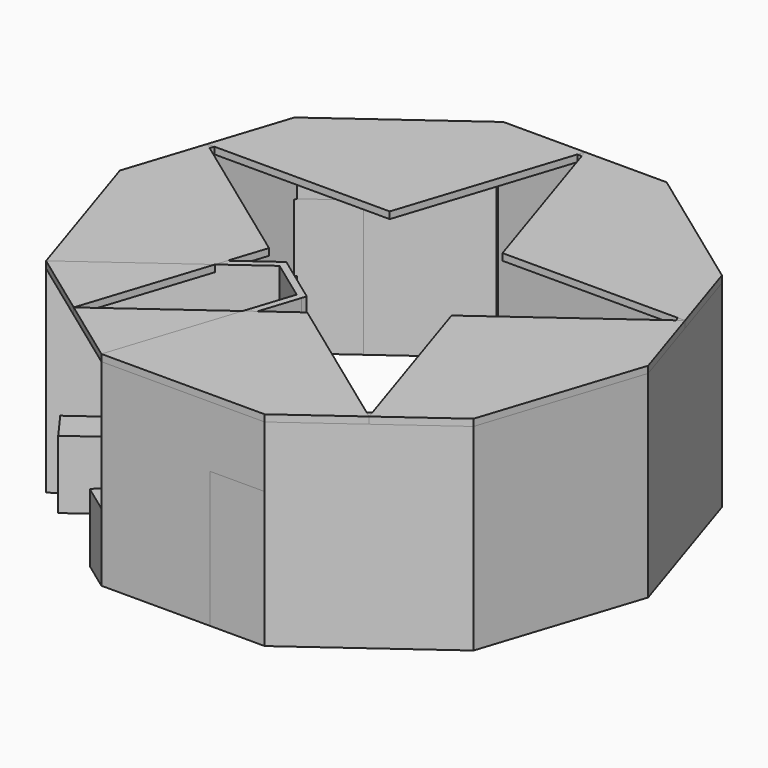
from build123d import *

# Parameters (mm, degrees)
F1_DEPTH     = 29.9999993294
F4_DEPTH     = 30
F6_DEPTH     = 10
F7_DEPTH     = 5
F9_DEPTH     = 30
F10_T        = 1
F10_T3_DEPTH = 32
F11_W        = 8
F11_H        = 20
F12_DEPTH    = 1.2370679775
F13_W        = 24
F13_H        = 10
F14_DEPTH    = 1.2370679775
F15_DEPTH    = 1
F17_DEPTH    = 1.2370679775
F18_DEPTH    = 1
F19_W        = 24
F19_H        = 29.9999993294
F20_DEPTH    = 1.2370679775
F21_DEPTH    = 1
F22_W        = 24
F22_H        = 10
F23_DEPTH    = 1.2370679775
F24_DEPTH    = 1
F25_DEPTH    = 1
F26_DEPTH    = 1
F28_DEPTH    = 1
F30_DEPTH    = 1
F31_DEPTH    = 1
F33_DEPTH    = 1
F34_DEPTH    = 10


# Not quite as in the source:
# - a shell that OpenCascade refuses in one call is made with other operations: the cavity is built on its own and cut out


with BuildPart() as f1:
    # F0 (on Top) → F1 (new body)
    with BuildSketch(Plane.XY):
        Polygon((31.416407865, 22.8253563911), (12, 36.9322024461), (-12, 36.9322024461), (-31.416407865, 22.8253563911), (-38.83281573, 0), (-31.416407865, -22.8253563911), (-12, -36.9322024461), (12, -36.9322024461), (31.416407865, -22.8253563911), (38.83281573, 0), align=None)
    extrude(amount=-F1_DEPTH)

    # F3 (on face) → F4 (cut)
    with BuildSketch(Plane.XY):
        Polygon((0, 0), (-31.416407865, -22.8253563911), (-12, -36.9322024461), align=None)
    extrude(amount=-F4_DEPTH, mode=Mode.SUBTRACT)

    # F8 (on face) → F9 (join)
    with BuildSketch(Plane.XY):
        Polygon((-3.7082039325, -11.4126781955), (0, 0), (-9.7082039325, -7.0534230275), align=None)
    extrude(amount=-F9_DEPTH)

    # F10: shell of thickness 1, made by hand


with BuildPart() as f6:
    # F5 (on face) → F6 (new body)
    with BuildSketch(Plane(origin=(0, 0, -29.9999993294), x_dir=(1, 0, 0), z_dir=(0, 0, -1))):
        with BuildLine():
            ThreePointArc((-16.0450849719, 33.9932761846), (-13.5450849719, 32.1769198646), (-10.4549150281, 32.1769198646))
            Line((-10.4549150281, 32.1769198646), (-12, 36.9322024461))
            Line((-12, 36.9322024461), (-16.0450849719, 33.9932761846))
        make_face()
    extrude(amount=-F6_DEPTH)


with BuildPart() as f7:
    # F5 (on face) → F7 (new body)
    with BuildSketch(Plane(origin=(0, 0, -29.9999993294), x_dir=(1, 0, 0), z_dir=(0, 0, -1))):
        Polygon((-19.3145152239, 23.8676935985), (-22.9290169684, 20.4129320816), (-16.0194939346, 13.1839285925), (-12.4049921901, 16.6386901094), align=None)
    extrude(amount=-F7_DEPTH)


with BuildPart() as f7b:
    # F5 (on face) → F7, piece 2 (new body)
    with BuildSketch(Plane(origin=(0, 0, -29.9999993294), x_dir=(1, 0, 0), z_dir=(0, 0, -1))):
        Polygon((-11.682091761, 17.3296424895), (-8.0675900164, 20.7844040064), (-14.9771131304, 28.0134074188), (-18.5916148367, 24.5586458618), align=None)
    extrude(amount=-F7_DEPTH)


with BuildPart() as f10_core1:
    # F10_t2: copy of F1
    add(f1.part)

    # the walls: a layer under each face that stays
    f10_faces = [f10_core1.faces().sort_by_distance(p)[0] for p in [
        (35.1246117975, -11.4126781955, -14.9999996647),
        (21.7082039325, -29.8787794186, -14.9999996647),
        (35.1246117975, 11.4126781955, -14.9999996647),
        (0, -36.9322024461, -14.9999996647),
        (21.7082039325, 29.8787794186, -14.9999996647),
        (-7.8541019662, -24.1724403208, -15),
        (-20.5623058987, -14.9393897093, -15),
        (-35.1246117975, -11.4126781955, -14.9999996647),
        (-35.1246117975, 11.4126781955, -14.9999996647),
        (-21.7082039325, 29.8787794186, -14.9999996647),
        (0, 36.9322024461, -14.9999996647),
        (-6.7082039325, -9.2330506115, -15),
    ]]
    thicken(f10_faces, amount=-F10_T, mode=Mode.SUBTRACT)

    # F10_s4 → F10_t3 (cut)
    with BuildSketch(Plane.XY.offset(-31)):
        Polygon((-3.7235923502, -11.4176781955), (-2.7571474162, -11.7216951899), (-2.5326334279, -11.0307121843), (-3.1204186802, -10.6036612012), align=None)
        Polygon((-9.7082039325, -7.0696033674), (-10.2959891848, -6.2444060331), (-9.7082039325, -5.81735505), (-9.1204186802, -6.2444060331), align=None)
    extrude(amount=F10_T3_DEPTH, mode=Mode.SUBTRACT)


with BuildPart() as f1_1:
    add(f1.part)

    # what is left inside the walls is the cavity
    f10_cavity = [f10_core1.part.solids().sort_by_distance(p)[0] for p in [
        (0, -11.977401, -0.01),
    ]]
    add(f10_cavity, mode=Mode.SUBTRACT)

    # F11 (on face) → F12 (cut, through all)
    with BuildSketch(Plane.XZ.offset(36.9322024461)):
        with Locations((8, -19.9999993294)):
            Rectangle(F11_W, F11_H)
    extrude(amount=-F12_DEPTH, mode=Mode.SUBTRACT)

    # F13 (on face) → F14 (cut, through all)
    with BuildSketch(Plane(origin=(-35.1246117975, 11.4126781955, 0), x_dir=(-0.3090169944, -0.9510565163, 0), z_dir=(-0.9510565163, 0.3090169944, 0))):
        with Locations((0, -24.9999993294)):
            Rectangle(F13_W, F13_H)
    extrude(amount=-F14_DEPTH, mode=Mode.SUBTRACT)

    # F16 (on face) → F17 (cut, through all)
    with BuildSketch(Plane(origin=(-21.7082039325, 29.8787794186, 0), x_dir=(-0.8090169944, -0.5877852523, 0), z_dir=(-0.5877852523, 0.8090169944, 0))):
        Polygon((4, -29.9999993294), (12, -29.9999993294), (12, -19.9999993294), (12, -9.9999993294), (4, -9.9999993294), align=None)
    extrude(amount=-F17_DEPTH, mode=Mode.SUBTRACT)

    # F19 (on face) → F20 (cut, through all)
    with BuildSketch(Plane(origin=(0, 36.9322024461, 0), x_dir=(-1, 0, 0), z_dir=(0, 1, 0))):
        with Locations((0, -14.9999996647)):
            Rectangle(F19_W, F19_H)
    extrude(amount=-F20_DEPTH, mode=Mode.SUBTRACT)

    # F22 (on face) → F23 (cut, through all)
    with BuildSketch(Plane(origin=(21.7082039325, 29.8787794186, 0), x_dir=(-0.8090169944, 0.5877852523, 0), z_dir=(0.5877852523, 0.8090169944, 0))):
        with Locations((0, -24.9999993294)):
            Rectangle(F22_W, F22_H)
    extrude(amount=-F23_DEPTH, mode=Mode.SUBTRACT)

    # F29 (on face) → F30 (cut)
    with BuildSketch(Plane(origin=(-35.1246117975, -11.4126781955, 0), x_dir=(0.3090169944, -0.9510565163, 0), z_dir=(-0.9510565163, -0.3090169944, 0))):
        Polygon((-12, -19.9999993294), (-12, -29.9999993294), (11, -30), (11, -4.9999993294), (-12, -4.9999993294), align=None)
    extrude(amount=-F30_DEPTH, mode=Mode.SUBTRACT)


with BuildPart() as f15:
    # F13 (on face) → F15 (new body)
    with BuildSketch(Plane(origin=(-35.1246117975, 11.4126781955, 0), x_dir=(-0.3090169944, -0.9510565163, 0), z_dir=(-0.9510565163, 0.3090169944, 0))):
        with Locations((0, -24.9999993294)):
            Rectangle(F13_W, F13_H)
    extrude(amount=-F15_DEPTH)


with BuildPart() as f18:
    # F16 (on face) → F18 (new body)
    with BuildSketch(Plane(origin=(-21.7082039325, 29.8787794186, 0), x_dir=(-0.8090169944, -0.5877852523, 0), z_dir=(-0.5877852523, 0.8090169944, 0))):
        Polygon((4, -29.9999993294), (12, -29.9999993294), (12, -19.9999993294), (12, -9.9999993294), (4, -9.9999993294), align=None)
    extrude(amount=-F18_DEPTH)


with BuildPart() as f21:
    # F19 (on face) → F21 (new body)
    with BuildSketch(Plane(origin=(0, 36.9322024461, 0), x_dir=(-1, 0, 0), z_dir=(0, 1, 0))):
        with Locations((0, -14.9999996647)):
            Rectangle(F19_W, F19_H)
    extrude(amount=-F21_DEPTH)


with BuildPart() as f24:
    # F22 (on face) → F24 (new body)
    with BuildSketch(Plane(origin=(21.7082039325, 29.8787794186, 0), x_dir=(-0.8090169944, 0.5877852523, 0), z_dir=(0.5877852523, 0.8090169944, 0))):
        with Locations((0, -24.9999993294)):
            Rectangle(F22_W, F22_H)
    extrude(amount=-F24_DEPTH)


with BuildPart() as f25:
    # F11 (on face) → F25 (new body)
    with BuildSketch(Plane.XZ.offset(36.9322024461)):
        with Locations((8, -19.9999993294)):
            Rectangle(F11_W, F11_H)
    extrude(amount=-F25_DEPTH)


with BuildPart() as f26:
    # F2 (on face) → F26 (new body)
    with BuildSketch(Plane.XY):
        Polygon((-8.2917960675, 11.4126781955), (0, 36.9322024461), (-12, 36.9322024461), (-31.416407865, 22.8253563911), (-35.1246117975, 11.4126781955), align=None)
    extrude(amount=-F26_DEPTH)


with BuildPart() as f26b:
    # F2 (on face) → F26, piece 2 (new body)
    with BuildSketch(Plane.XY):
        Polygon((12, 36.9322024461), (0, 36.9322024461), (8.2917960675, 11.4126781955), (35.1246117975, 11.4126781955), (31.416407865, 22.8253563911), align=None)
    extrude(amount=-F26_DEPTH)


with BuildPart() as f26c:
    # F2 (on face) → F26, piece 3 (new body)
    with BuildSketch(Plane.XY):
        Polygon((38.83281573, 0), (35.1246117975, 11.4126781955), (13.416407865, -4.359255168), (21.7082039325, -29.8787794186), (31.416407865, -22.8253563911), align=None)
    extrude(amount=-F26_DEPTH)


with BuildPart() as f28:
    # F27 (on face) → F28 (new body)
    with BuildSketch(Plane.XY):
        Polygon((-38.83281573, 0), (-31.416407865, -22.8253563911), (-15.7082039325, -11.4126781955), (-13.416407865, -4.359255168), (-35.1246117975, 11.4126781955), align=None)
    extrude(amount=-F28_DEPTH)


with BuildPart() as f28b:
    # F27 (on face) → F28, piece 2 (new body)
    with BuildSketch(Plane.XY):
        Polygon((-6, -18.4661012231), (-12, -36.9322024461), (12, -36.9322024461), (21.7082039325, -29.8787794186), (0, -14.106846055), align=None)
    extrude(amount=-F28_DEPTH)


with BuildPart() as f31:
    # F29 (on face) → F31 (new body)
    with BuildSketch(Plane(origin=(-35.1246117975, -11.4126781955, 0), x_dir=(0.3090169944, -0.9510565163, 0), z_dir=(-0.9510565163, -0.3090169944, 0))):
        Polygon((-12, -4.9999993294), (-12, -29.9999993294), (11, -30), (11, -4.9999993294), align=None)
    extrude(amount=-F31_DEPTH)


with BuildPart() as f33:
    # F32 (on face) → F33 (new body)
    with BuildSketch(Plane.XY):
        Polygon((-15.7082039325, -11.4126781955), (-31.416407865, -22.8253563911), (-21.7082039325, -29.8787794186), align=None)
    extrude(amount=-F33_DEPTH)


with BuildPart() as f33b:
    # F32 (on face) → F33, piece 2 (new body)
    with BuildSketch(Plane.XY):
        Polygon((-6, -18.4661012231), (-21.7082039325, -29.8787794186), (-12, -36.9322024461), align=None)
    extrude(amount=-F33_DEPTH)


with BuildPart() as f34:
    # F5 (on face) → F34 (new body)
    with BuildSketch(Plane(origin=(0, 0, -29.9999993294), x_dir=(1, 0, 0), z_dir=(0, 0, -1))):
        Polygon((-27.1631538232, 25.9155263348), (-30.1020800847, 21.870441363), (-25.2479781185, 18.3437298492), (-22.309051857, 22.3888148211), align=None)
    extrude(amount=-F34_DEPTH)


solid = Compound([f6.part, f7.part, f7b.part, f1_1.part, f15.part, f18.part, f21.part, f24.part, f25.part, f26.part, f26b.part, f26c.part, f28.part, f28b.part, f31.part, f33.part, f33b.part, f34.part])
